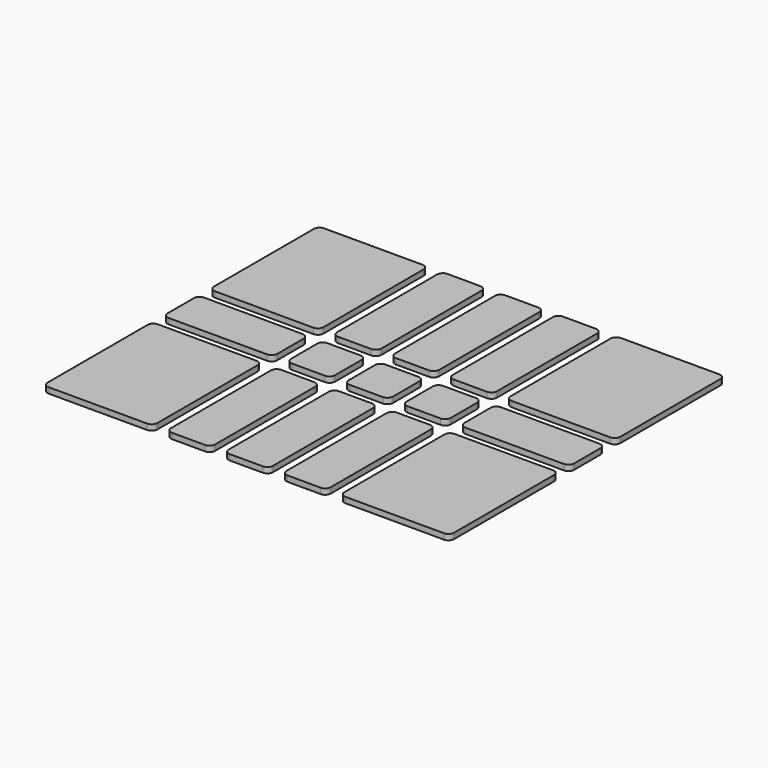
from build123d import *

# Parameters (mm, degrees)
F1_DEPTH = 1


with BuildPart() as f1:
    # F0 (on Top) → F1 (new body)
    with BuildSketch(Plane.XY):
        with BuildLine():
            Line((-17.5, -6.3), (-34.85, -6.3))
            ThreePointArc((-34.85, -6.3), (-35.5571067812, -6.5928932188), (-35.85, -7.3))
            Line((-35.85, -7.3), (-35.85, -29.35))
            ThreePointArc((-35.85, -29.35), (-35.5571067812, -30.0571067812), (-34.85, -30.35))
            Line((-34.85, -30.35), (-17.5, -30.35))
            ThreePointArc((-17.5, -30.35), (-16.7928932188, -30.0571067812), (-16.5, -29.35))
            Line((-16.5, -29.35), (-16.5, -7.3))
            ThreePointArc((-16.5, -7.3), (-16.7928932188, -6.5928932188), (-17.5, -6.3))
        make_face()
    extrude(amount=F1_DEPTH)


with BuildPart() as f1b:
    # F0 (on Top) → F1, piece 2 (new body)
    with BuildSketch(Plane.XY):
        with BuildLine():
            Line((-7.3, -6.3), (-13.1, -6.3))
            ThreePointArc((-13.1, -6.3), (-13.8071067812, -6.5928932188), (-14.1, -7.3))
            Line((-14.1, -7.3), (-14.1, -29.35))
            ThreePointArc((-14.1, -29.35), (-13.8071067812, -30.0571067812), (-13.1, -30.35))
            Line((-13.1, -30.35), (-7.3, -30.35))
            ThreePointArc((-7.3, -30.35), (-6.5928932188, -30.0571067812), (-6.3, -29.35))
            Line((-6.3, -29.35), (-6.3, -7.3))
            ThreePointArc((-6.3, -7.3), (-6.5928932188, -6.5928932188), (-7.3, -6.3))
        make_face()
    extrude(amount=F1_DEPTH)


with BuildPart() as f1c:
    # F0 (on Top) → F1, piece 3 (new body)
    with BuildSketch(Plane.XY):
        with BuildLine():
            Line((2.9, -6.3), (-2.9, -6.3))
            ThreePointArc((-2.9, -6.3), (-3.6071067812, -6.5928932188), (-3.9, -7.3))
            Line((-3.9, -7.3), (-3.9, -29.35))
            ThreePointArc((-3.9, -29.35), (-3.6071067812, -30.0571067812), (-2.9, -30.35))
            Line((-2.9, -30.35), (2.9, -30.35))
            ThreePointArc((2.9, -30.35), (3.6071067812, -30.0571067812), (3.9, -29.35))
            Line((3.9, -29.35), (3.9, -7.3))
            ThreePointArc((3.9, -7.3), (3.6071067812, -6.5928932188), (2.9, -6.3))
        make_face()
    extrude(amount=F1_DEPTH)


with BuildPart() as f1d:
    # F0 (on Top) → F1, piece 4 (new body)
    with BuildSketch(Plane.XY):
        with BuildLine():
            Line((-17.5, 3.9), (-34.85, 3.9))
            ThreePointArc((-34.85, 3.9), (-35.5571067812, 3.6071067812), (-35.85, 2.9))
            Line((-35.85, 2.9), (-35.85, -2.9))
            ThreePointArc((-35.85, -2.9), (-35.5571067812, -3.6071067812), (-34.85, -3.9))
            Line((-34.85, -3.9), (-17.5, -3.9))
            ThreePointArc((-17.5, -3.9), (-16.7928932188, -3.6071067812), (-16.5, -2.9))
            Line((-16.5, -2.9), (-16.5, 2.9))
            ThreePointArc((-16.5, 2.9), (-16.7928932188, 3.6071067812), (-17.5, 3.9))
        make_face()
    extrude(amount=F1_DEPTH)



with BuildPart() as f1e:
    # F0 (on Top) → F1, piece 5 (new body)
    with BuildSketch(Plane.XY):
        with BuildLine():
            Line((-7.3, 3.9), (-13.1, 3.9))
            ThreePointArc((-13.1, 3.9), (-13.8071067812, 3.6071067812), (-14.1, 2.9))
            Line((-14.1, 2.9), (-14.1, -2.9))
            ThreePointArc((-14.1, -2.9), (-13.8071067812, -3.6071067812), (-13.1, -3.9))
            Line((-13.1, -3.9), (-7.3, -3.9))
            ThreePointArc((-7.3, -3.9), (-6.5928932188, -3.6071067812), (-6.3, -2.9))
            Line((-6.3, -2.9), (-6.3, 2.9))
            ThreePointArc((-6.3, 2.9), (-6.5928932188, 3.6071067812), (-7.3, 3.9))
        make_face()
    extrude(amount=F1_DEPTH)


with BuildPart() as f1f:
    # F0 (on Top) → F1, piece 6 (new body)
    with BuildSketch(Plane.XY):
        with BuildLine():
            Line((2.9, 3.9), (-2.9, 3.9))
            ThreePointArc((-2.9, 3.9), (-3.6071067812, 3.6071067812), (-3.9, 2.9))
            Line((-3.9, 2.9), (-3.9, -2.9))
            ThreePointArc((-3.9, -2.9), (-3.6071067812, -3.6071067812), (-2.9, -3.9))
            Line((-2.9, -3.9), (2.9, -3.9))
            ThreePointArc((2.9, -3.9), (3.6071067812, -3.6071067812), (3.9, -2.9))
            Line((3.9, -2.9), (3.9, 2.9))
            ThreePointArc((3.9, 2.9), (3.6071067812, 3.6071067812), (2.9, 3.9))
        make_face()
    extrude(amount=F1_DEPTH)


with BuildPart() as f1d_1:
    add(f1d.part)

    add(f1e.part)  # F2 merges F1e

    add(f1f.part)  # F2 merges F1f
    # F2: F1, F1b, F1c, F1d, F1e, F1f across plane
    add(f1.part.mirror(Plane.XZ))
    add(f1b.part.mirror(Plane.XZ))
    add(f1c.part.mirror(Plane.XZ))
    add(f1d.part.mirror(Plane.XZ))
    add(f1e.part.mirror(Plane.XZ))
    add(f1f.part.mirror(Plane.XZ))


with BuildPart() as f1c_1:
    add(f1c.part)

    add(f1d_1.part)  # F3 merges F1d
    # F3: F1, F1b, F1c, F1d across plane
    add(f1.part.mirror(Plane.YZ))
    add(f1b.part.mirror(Plane.YZ))
    add(f1c.part.mirror(Plane.YZ))
    add(f1d_1.part.mirror(Plane.YZ))


solid = Compound([f1.part, f1b.part, f1c_1.part])
